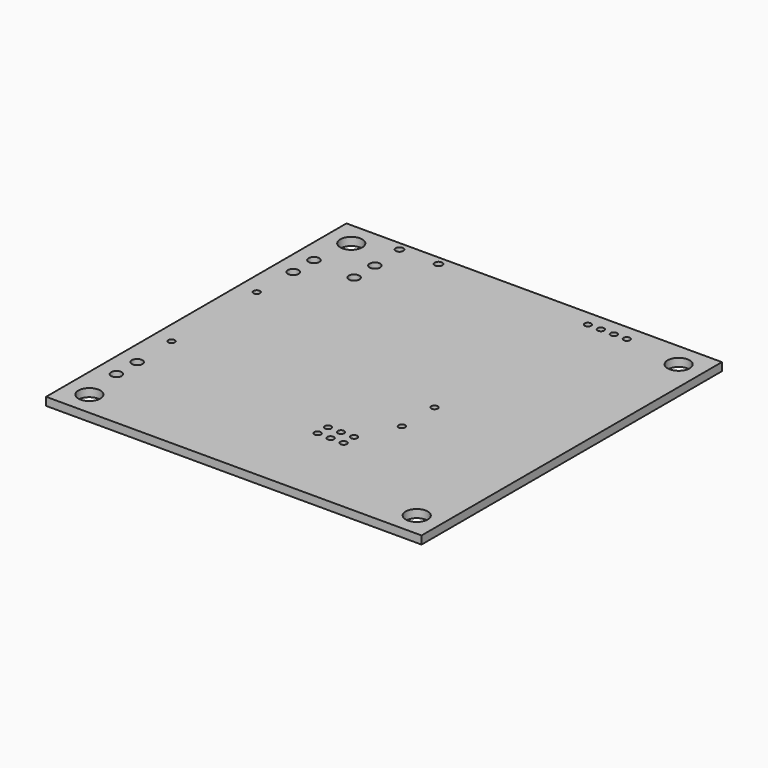
from build123d import *

# Parameters (mm, degrees)
F0_W            = 73.4
F0_H            = 73.4
F0_R            = 2.15
F1_DEPTH        = 1.5748
F2_R            = 0.635
F3_DEPTH        = 1.5758
F4_W            = 5
F4_H            = 5
F5_DEPTH        = 0.0508
F5_COPIES_COUNT = 24
F8_R            = 0.74
F9_DEPTH        = 1.5758
F10_R           = 1.038
F11_DEPTH       = 1.5758
F7_R            = 1.016
F12_DEPTH       = 1.524
F13_R           = 0.635
F14_DEPTH       = 1.5758
F15_R           = 0.635
F16_DEPTH       = 1.5758


# Not quite as in the source:
# - a pattern or mirror of a feature is missing from the dataset's text; its kind, count and spacing are read off the source's solid


with BuildPart() as f1:
    # F0 (on Top) → F1 (new body)
    with BuildSketch(Plane.XY):
        Rectangle(F0_W, F0_H)
        with Locations((-32, -32)):
            Circle(F0_R, mode=Mode.SUBTRACT)
        with Locations((32, -32)):
            Circle(F0_R, mode=Mode.SUBTRACT)
        with Locations((-32, 32)):
            Circle(F0_R, mode=Mode.SUBTRACT)
        with Locations((32, 32)):
            Circle(F0_R, mode=Mode.SUBTRACT)
    extrude(amount=F1_DEPTH)

    # F2 (on Top) → F3 (cut, through all)
    with BuildSketch(Plane.XY):
        with Locations((-33.2, -10.4)):
            Circle(F2_R)
        with Locations((-33.2, 10.4)):
            Circle(F2_R)
        with Locations((11.8, -10.4)):
            Circle(F2_R)
        with Locations((11.8, -2.4)):
            Circle(F2_R)
    extrude(amount=F3_DEPTH, mode=Mode.SUBTRACT)

    # F4 (on face) → F5 (join)
    with BuildSketch(Plane(origin=(0, 0, 0), x_dir=(1, 0, 0), z_dir=(0, 0, -1))):
        with Locations((29.53, 0)):
            Rectangle(F4_W, F4_H)
    f5 = extrude(amount=F5_DEPTH)

    # F5_copies: F5 ×24 about axis
    f5_copies_axis = Axis((0, 0, 0), (0, 0, 1))
    for i in range(1, F5_COPIES_COUNT):
        add(f5.rotate(f5_copies_axis, i * 360 / F5_COPIES_COUNT))

    # F8 (on Top) → F9 (cut, through all)
    with BuildSketch(Plane.XY):
        with Locations((-24.97, 35)):
            Circle(F8_R)
        with Locations((-17.35, 35)):
            Circle(F8_R)
    extrude(amount=F9_DEPTH, mode=Mode.SUBTRACT)

    # F10 (on Top) → F11 (cut, through all)
    with BuildSketch(Plane.XY):
        with Locations((-24.6, 28.53)):
            Circle(F10_R)
        with Locations((-24.6, 23.45)):
            Circle(F10_R)
        with Locations((-33, 24.14)):
            Circle(F10_R)
        with Locations((-33, 19.06)):
            Circle(F10_R)
        with Locations((-33, -19.06)):
            Circle(F10_R)
        with Locations((-33, -24.14)):
            Circle(F10_R)
    extrude(amount=F11_DEPTH, mode=Mode.SUBTRACT)

    # F7 (on Top) → F12 (cut)
    with BuildSketch(Plane.XY):
        Circle(F7_R)
    extrude(amount=F12_DEPTH, mode=Mode.SUBTRACT)

    # F13 (on Top) → F14 (cut, through all)
    with BuildSketch(Plane.XY):
        with Locations((12.98, 33.6)):
            Circle(F13_R)
        with Locations((15.52, 33.6)):
            Circle(F13_R)
        with Locations((18.06, 33.6)):
            Circle(F13_R)
        with Locations((20.6, 33.6)):
            Circle(F13_R)
    extrude(amount=F14_DEPTH, mode=Mode.SUBTRACT)

    # F15 (on Top) → F16 (cut, through all)
    with BuildSketch(Plane.XY):
        with Locations((3.22, -17.7)):
            Circle(F15_R)
        with Locations((3.22, -20.24)):
            Circle(F15_R)
        with Locations((5.76, -20.24)):
            Circle(F15_R)
        with Locations((5.76, -17.7)):
            Circle(F15_R)
        with Locations((8.3, -17.7)):
            Circle(F15_R)
        with Locations((8.3, -20.24)):
            Circle(F15_R)
    extrude(amount=F16_DEPTH, mode=Mode.SUBTRACT)


solid = f1.part
